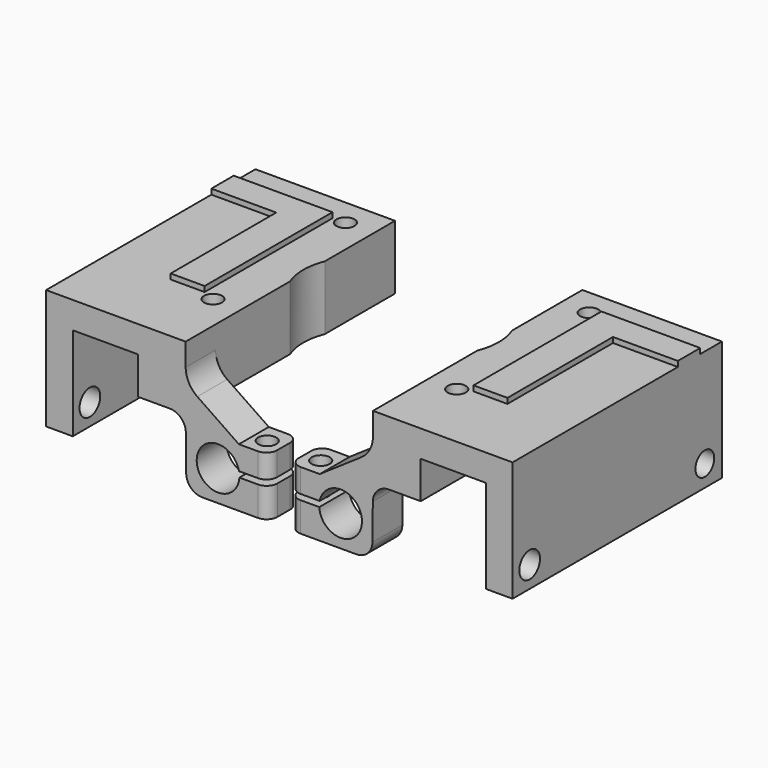
from build123d import *

# Parameters (mm, degrees)
F1_DEPTH      = 7
F2_DEPTH      = 42
F3_R          = 1.7
F3_R_2        = 11
F4_DEPTH      = 12.001
F5_R          = 4
F6_DEPTH      = 10
F7_DEPTH      = 12.001
F8_R          = 1.4
F9_DEPTH      = 10.9920075553
F8_R_2        = 1.7
F10_DEPTH     = 4.4348209087
F11_R         = 5
F12_R         = 3
F13_R         = 3
F14_R         = 2
F15_R         = 2.2
F15_R_2       = 2.4255023423
F16_DEPTH     = 6
F17_TEXT_SIZE = 41.9437823343
F18_DEPTH     = 1


# Not quite as in the source:
# - a feature names something its author has since deleted; it is built from what else it names
# - Text() gives the source's letters only with a copy of the font that has no kerning and outlines rounded to 1/6400 em; it was checked with that copy


with BuildPart() as f1:
    # F0 (on Front) → F1 (new body)
    with BuildSketch(Plane.XZ):
        Polygon((-18.6721007523, 29.8099789735), (-18.6721007523, 7.3259699669), (-13.6721007523, 7.3259699669), (-13.6721007523, 24.8099789735), (-1.4721007523, 24.8099789735), (-1.4721007523, 17.8099789735), (7.4637966118, 17.8099789735), (7.4637966118, 22.9406704692), (7.4637966118, 29.8099789735), align=None)
        Polygon((17.4301751077, 16.1394868046), (7.4637966118, 22.9406704692), (7.4637966118, 17.8099789735), (7.5940201178, 5.1484792493), (23.0186601057, 5.1484792493), (23.0186601057, 10.6682249423), (15.6860510706, 10.6682249423), (15.6860510706, 11.7046658959), (22.9896428882, 11.7046658959), (22.9896428882, 16.1394868046), align=None)
    extrude(amount=F1_DEPTH)

    # F0 (on Front) → F2 (join)
    with BuildSketch(Plane.XZ):
        Polygon((-18.6721007523, 29.8099789735), (-18.6721007523, 7.3259699669), (-13.6721007523, 7.3259699669), (-13.6721007523, 24.8099789735), (-1.4721007523, 24.8099789735), (-1.4721007523, 17.8099789735), (7.4637966118, 17.8099789735), (7.4637966118, 22.9406704692), (7.4637966118, 29.8099789735), align=None)
    extrude(amount=-F2_DEPTH)

    # F3 (on face) → F4 (cut, through all)
    with BuildSketch(Plane(origin=(0, 0, 17.8099789735), x_dir=(1, 0, 0), z_dir=(0, 0, -1))):
        with Locations((2.1850741468, -6)):
            Circle(F3_R)
        with Locations((2.1850741468, -37)):
            Circle(F3_R)
        with Locations((17.6850741468, -21.5)):
            Circle(F3_R_2)
    extrude(amount=-F4_DEPTH, mode=Mode.SUBTRACT)

    # F5 (on face) → F6 (cut)
    with BuildSketch(Plane.XZ.offset(7)):
        with Locations((13.5278992477, 10.8989789735)):
            Circle(F5_R)
    extrude(amount=-F6_DEPTH, mode=Mode.SUBTRACT)

    # F3 (on face) → F7 (cut, through all)
    with BuildSketch(Plane(origin=(0, 0, 17.8099789735), x_dir=(1, 0, 0), z_dir=(0, 0, -1))):
        with Locations((2.1850741468, -6)):
            Circle(F3_R)
        with Locations((2.1850741468, -37)):
            Circle(F3_R)
        with Locations((17.6850741468, -21.5)):
            Circle(F3_R_2)
    extrude(amount=-F7_DEPTH, mode=Mode.SUBTRACT)

    # F8 (on face) → F9 (cut, through all)
    with BuildSketch(Plane.XY.offset(16.1394868046)):
        with Locations((19.9896428882, -3.5767070949)):
            Circle(F8_R)
    extrude(amount=-F9_DEPTH, mode=Mode.SUBTRACT)

    # F8 (on face) → F10 (cut, through all)
    with BuildSketch(Plane.XY.offset(16.1394868046)):
        with Locations((19.9896428882, -3.5767070949)):
            Circle(F8_R_2)
        with Locations((19.9896428882, -3.5767070949)):
            Circle(F8_R, mode=Mode.SUBTRACT)
    extrude(amount=-F10_DEPTH, mode=Mode.SUBTRACT)

    # F11
    f11_edges = [f1.edges().sort_by_distance(p)[0] for p in [
        (7.463797, -3.5, 22.94067),
    ]]
    fillet(f11_edges, radius=F11_R)

    # F12
    f12_edges = [f1.edges().sort_by_distance(p)[0] for p in [
        (7.463797, -3.5, 17.809979),
    ]]
    fillet(f12_edges, radius=F12_R)

    # F13
    f13_edges = [f1.edges().sort_by_distance(p)[0] for p in [
        (7.59402, -3.5, 5.148479),
    ]]
    fillet(f13_edges, radius=F13_R)

    # F14
    f14_edges = [f1.edges().sort_by_distance(p)[0] for p in [
        (22.989643, -7, 13.922076),
        (23.01866, -7, 7.908352),
        (22.989643, 0, 13.922076),
        (23.01866, 0, 7.908352),
    ]]
    fillet(f14_edges, radius=F14_R)

    # F15 (on face) → F16 (cut)
    with BuildSketch(Plane(origin=(-18.6721007523, 0, 0), x_dir=(0, -1, 0), z_dir=(-1, 0, 0))):
        with Locations((-38, 11.3259699669)):
            Circle(F15_R)
        with Locations((3, 11.3259699669)):
            Circle(F15_R_2)
    extrude(amount=-F16_DEPTH, mode=Mode.SUBTRACT)

    # F17 (on face) → F18 (join)
    with BuildSketch(Plane.XY.offset(29.8099789735)):
        with Locations(Location((3.5908724648, 36.9253193088), (0, 0, 180))):
            Text('L', F17_TEXT_SIZE, font='Open Sans', font_style=FontStyle.BOLD, text_align=(TextAlign.LEFT, TextAlign.BOTTOM))
    extrude(amount=F18_DEPTH)


with BuildPart() as f19_1:
    # F19: instance of F1
    add(f1.part.mirror(Plane.YZ))


with BuildPart() as f19_1_1:
    # F20: moved
    add(f19_1.part.moved(Location((50, 0, 0))))


solid = Compound([f1.part, f19_1_1.part])
